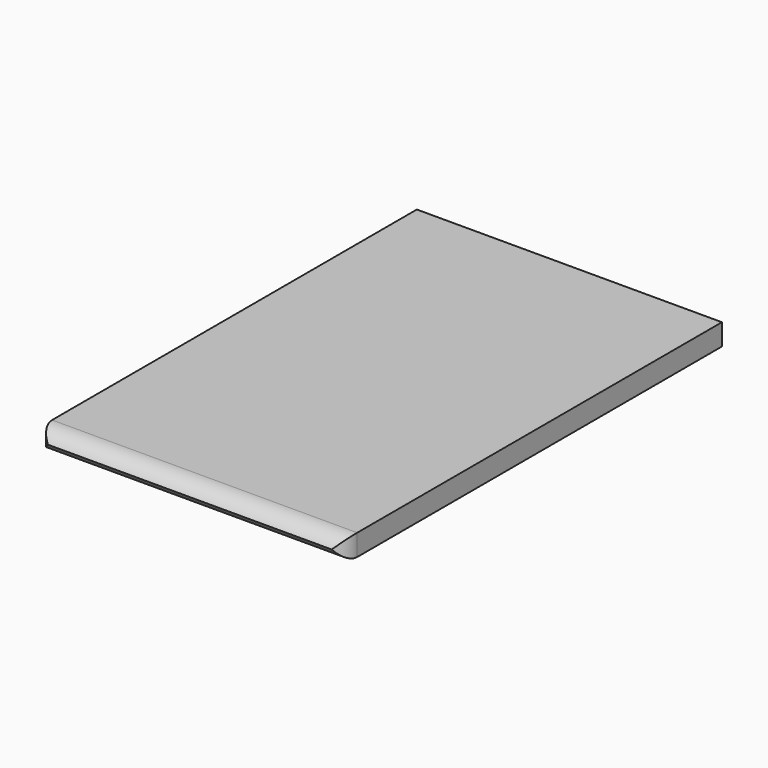
from build123d import *

# Parameters (mm, degrees)
F0_W        = 36.2067520618
F0_H        = 56.6427242011
F1_DEPTH    = 2.54
F2_T1_DEPTH = 15.24
F2_T3_DEPTH = 48.9067520618


# Not quite as in the source:
# - a fillet or chamfer that OpenCascade refuses, or shapes differently, is made with other operations: its cross-section is extruded or revolved along the edge and cut away or added


with BuildPart() as f1:
    # F0 (on Top) → F1 (new body)
    with BuildSketch(Plane.XY):
        with Locations((-102.4080365896, -10.3280926123)):
            Rectangle(F0_W, F0_H)
    extrude(amount=F1_DEPTH)

    # F2: fillet of radius 2.54 on 4 edges, made by hand

    # F2_s2 → F2_t1 (cut)
    with BuildSketch(Plane.XY.offset(-6.35)):
        with BuildLine():
            ThreePointArc((-120.5114126205, -36.1094547129), (-119.7674638448, -37.9055059371), (-117.9714126205, -38.6494547129))
            Line((-117.9714126205, -38.6494547129), (-120.5114126205, -38.6494547129))
            Line((-120.5114126205, -38.6494547129), (-120.5114126205, -36.1094547129))
        make_face()
        with BuildLine():
            ThreePointArc((-86.8446605587, -38.6494547129), (-85.0486093345, -37.9055059371), (-84.3046605587, -36.1094547129))
            Line((-84.3046605587, -36.1094547129), (-84.3046605587, -38.6494547129))
            Line((-84.3046605587, -38.6494547129), (-86.8446605587, -38.6494547129))
        make_face()
    extrude(amount=F2_T1_DEPTH, mode=Mode.SUBTRACT)

    # F2_s4 → F2_t3 (cut)
    with BuildSketch(Plane.YZ.offset(-126.8614126205)):
        with BuildLine():
            ThreePointArc((-38.6494547129, 2.54), (-37.9055059371, 0.7439487758), (-36.1094547129, 0))
            Line((-36.1094547129, 0), (-38.6494547129, 0))
            Line((-38.6494547129, 0), (-38.6494547129, 2.54))
        make_face()
        with BuildLine():
            ThreePointArc((-38.6494547129, 0), (-37.9055059371, 1.7960512242), (-36.1094547129, 2.54))
            Line((-36.1094547129, 2.54), (-38.6494547129, 2.54))
            Line((-38.6494547129, 2.54), (-38.6494547129, 0))
        make_face()
    extrude(amount=F2_T3_DEPTH, mode=Mode.SUBTRACT)


solid = f1.part
